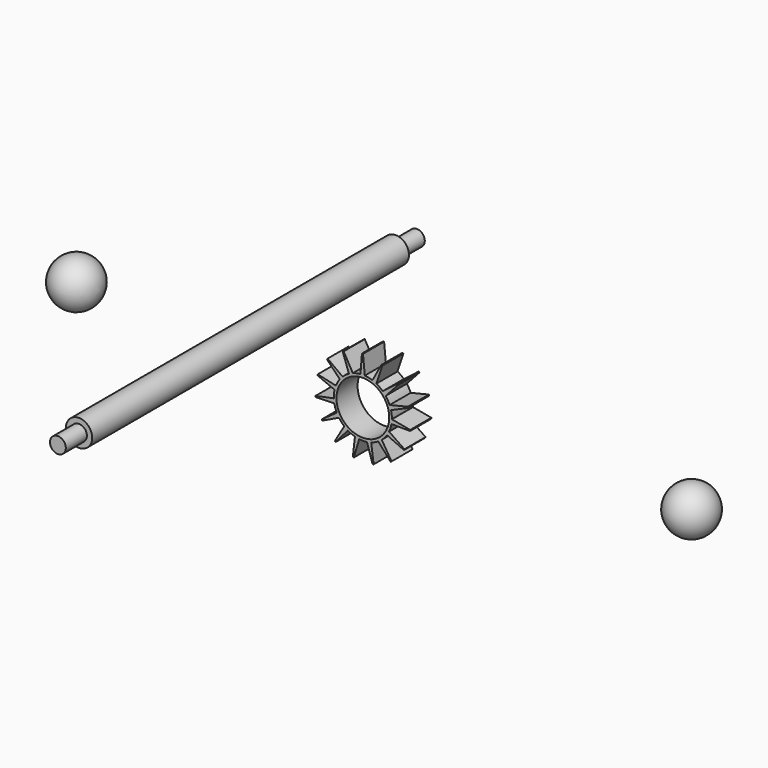
from build123d import *

# Parameters (mm, degrees)
F1_DEPTH        = 5
F1_COPIES_COUNT = 15
F3_R            = 5
F4_DEPTH        = 25
F5_R            = 2.5
F6_DEPTH        = 37.5
F7_R            = 1.5
F8_DEPTH        = 5
F12_DEPTH       = 5


# Not quite as in the source:
# - a feature of the source that left no trace in its solid (it failed there, or was rolled back) is left out
# - a pattern or mirror of a feature is missing from the dataset's text; its kind, count and spacing are read off the source's solid


with BuildPart() as f1:
    # F0 (on Front) → F1 (new body)
    with BuildSketch(Plane.XZ):
        with BuildLine():
            ThreePointArc((-0.4480475583, 5.4817199295), (-3.727313941, -4.0443949838), (5.5, 0))
            ThreePointArc((5.5, 0), (4.0167616325, 3.7570767876), (0.3670450953, 5.4877388693))
            ThreePointArc((0.3670450953, 5.4877388693), (-0.0406128879, 5.4998500519), (-0.4480475583, 5.4817199295))
        make_face()
        with BuildLine():
            ThreePointArc((-0.4480475583, 5.4817199295), (-0.0406128879, 5.4998500519), (0.3670450953, 5.4877388693))
            Line((0.3670450953, 5.4877388693), (0.02510037, 9))
            Line((0.02510037, 9), (-0.17489963, 9))
            Line((-0.17489963, 9), (-0.4480475583, 5.4817199295))
        make_face()
    extrude(amount=F1_DEPTH)

    # F1_copies: F1 ×15 about axis
    f1_copies_axis = Axis((0, 0, 0), (0, 1, 0))


with BuildPart() as f1_1:
    add(f1.part)
    for i in range(1, F1_COPIES_COUNT):
        add(f1.part.rotate(f1_copies_axis, i * 360 / F1_COPIES_COUNT))

    # F3 (on face) → F4 (cut)
    with BuildSketch(Plane.XZ.offset(5)):
        Circle(F3_R)
    extrude(amount=-F4_DEPTH, mode=Mode.SUBTRACT)


with BuildPart() as f6:
    # F5 (on Front) → F6 (new body, symmetric)
    with BuildSketch(Plane.XZ):
        with Locations((-27.7663727778, 0)):
            Circle(F5_R)
    extrude(amount=F6_DEPTH, both=True)

    # F7 (on face) → F8 (join)
    with BuildSketch(Plane.XZ.offset(37.5)):
        with Locations((-27.7663727778, 0)):
            Circle(F7_R)
    extrude(amount=F8_DEPTH)

    # F9: F6 across plane


with BuildPart() as f6_1:
    add(f6.part)
    add(f6.part.mirror(Plane.XZ))


with BuildPart() as f11:
    # F10 (on Top) → F11 (revolve)
    with BuildSketch(Plane.XY):
        with BuildLine():
            Line((-58.2629402318, 0), (-58.2629402318, -4.5))
            ThreePointArc((-58.2629402318, -4.5), (-53.8277467134, -0.7609589043), (-56.7629402318, 4.2426406871))
            Line((-56.7629402318, 4.2426406871), (-58.2629402318, 4.2426406871))
            Line((-58.2629402318, 4.2426406871), (-58.2629402318, 0))
        make_face()
    revolve(axis=Axis((-58.2629402318, -2.25, 0), (0, -1, 0)))

    # F12 (cut): a face of the model
    f12_faces = [f11.faces().sort_by_distance(p)[0] for p in [
        (-58.2629402318, 4.2426406871, 0),
    ]]
    extrude(f12_faces, amount=-F12_DEPTH, mode=Mode.SUBTRACT)


with BuildPart() as f13_1:
    # F13: instance of F11
    add(f11.part.mirror(Plane.YZ))


solid = Compound([f1_1.part, f6_1.part, f11.part, f13_1.part])
